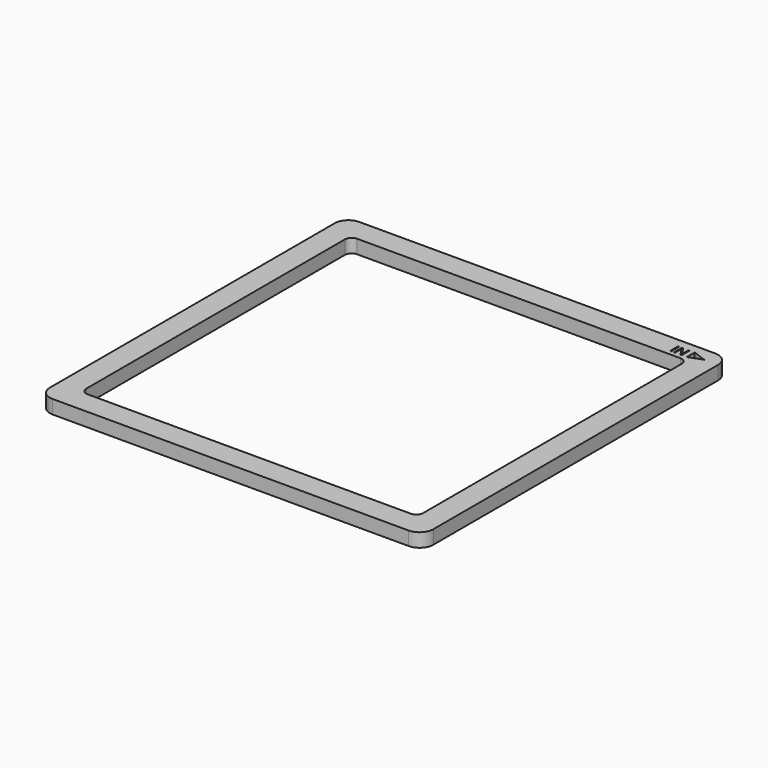
from build123d import *

# Parameters (mm, degrees)
F1_DEPTH     = 10
F3_TEXT_SIZE = 10.1102842852
F4_DEPTH     = 10.001


# Not quite as in the source:
# - Text() gives the source's letters only with a copy of the font that has no kerning and outlines rounded to 1/6400 em; it was checked with that copy


with BuildPart() as f1:
    # F0 (on Top) → F1 (new body)
    with BuildSketch(Plane.XY):
        with BuildLine():
            ThreePointArc((140, 130), (137.0710678119, 137.0710678119), (130, 140))
            Line((130, 140), (-130, 140))
            ThreePointArc((-130, 140), (-137.0710678119, 137.0710678119), (-140, 130))
            Line((-140, 130), (-140, -130))
            ThreePointArc((-140, -130), (-137.0710678119, -137.0710678119), (-130, -140))
            Line((-130, -140), (130, -140))
            ThreePointArc((130, -140), (137.0710678119, -137.0710678119), (140, -130))
            Line((140, -130), (140, 130))
        make_face()
    extrude(amount=F1_DEPTH)

    # F3 (on face) + F1_face1 (on face) → F4 (cut, through all)
    with BuildSketch(Plane.XY.offset(10)):
        Polygon((120, 126.3602976573), (130, 130), (120, 133.6397023427), align=None)
        with BuildLine():
            Line((118, 123), (-118, 123))
            ThreePointArc((-118, 123), (-121.5355339059, 121.5355339059), (-123, 118))
            Line((-123, 118), (-123, -118))
            ThreePointArc((-123, -118), (-121.5355339059, -121.5355339059), (-118, -123))
            Line((-118, -123), (118, -123))
            ThreePointArc((118, -123), (121.5355339059, -121.5355339059), (123, -118))
            Line((123, -118), (123, 118))
            ThreePointArc((123, 118), (121.5355339059, 121.5355339059), (118, 123))
        make_face()
        with Locations((106.8960346425, 126.3602976573)):
            Text('IN', F3_TEXT_SIZE, font='Open Sans', text_align=(TextAlign.LEFT, TextAlign.BOTTOM))
    with BuildSketch(Plane(origin=(0, 0, 0), x_dir=(1, 0, 0), z_dir=(0, 0, -1))):
        with BuildLine():
            ThreePointArc((130, -140), (137.0710678119, -137.0710678119), (140, -130))
            Line((140, -130), (140, 130))
            ThreePointArc((140, 130), (137.0710678119, 137.0710678119), (130, 140))
            Line((130, 140), (-130, 140))
            ThreePointArc((-130, 140), (-137.0710678119, 137.0710678119), (-140, 130))
            Line((-140, 130), (-140, -130))
            ThreePointArc((-140, -130), (-137.0710678119, -137.0710678119), (-130, -140))
            Line((-130, -140), (130, -140))
        make_face()
    extrude(amount=-F4_DEPTH, dir=(0, 0, 1), mode=Mode.SUBTRACT)


solid = f1.part
